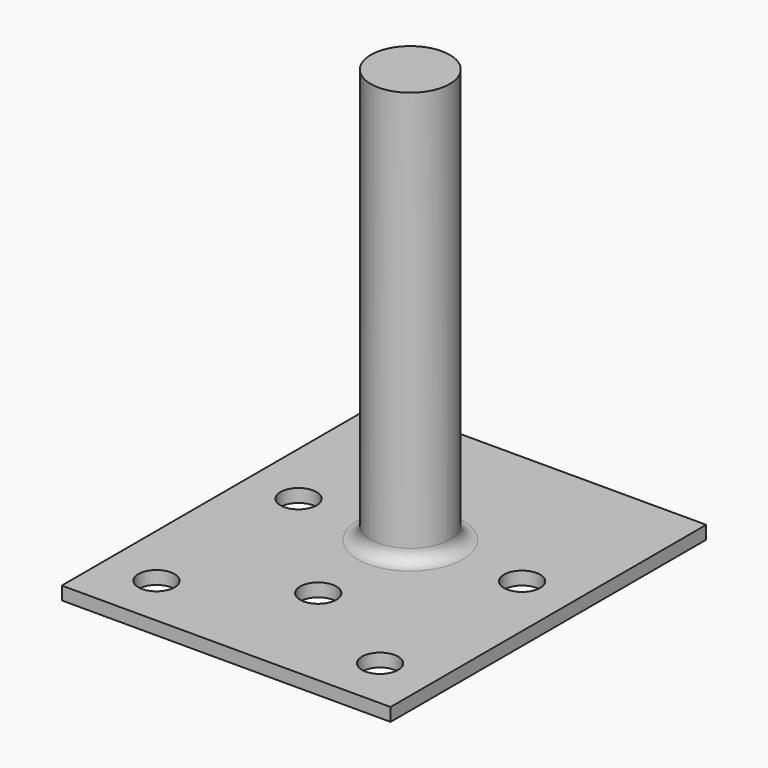
from build123d import *

# Parameters (mm, degrees)
F0_R     = 5.5
F0_R_2   = 12
F1_DEPTH = 4
F2_R     = 12
F3_DEPTH = 130
F4_R     = 4


with BuildPart() as f1:
    # F0 (on Top) → F1 (new body)
    with BuildSketch(Plane.XY):
        Polygon((50, 50), (0, 50), (-50, 50), (-50, -70), (0, -70), (50, -70), align=None)
        with Locations((-34, -54)):
            Circle(F0_R, mode=Mode.SUBTRACT)
        with Locations((34, -54)):
            Circle(F0_R, mode=Mode.SUBTRACT)
        with Locations((0, -35)):
            Circle(F0_R, mode=Mode.SUBTRACT)
        with Locations((-34, 0)):
            Circle(F0_R, mode=Mode.SUBTRACT)
        Circle(F0_R_2, mode=Mode.SUBTRACT)
        with Locations((34, 0)):
            Circle(F0_R, mode=Mode.SUBTRACT)
    extrude(amount=F1_DEPTH)

    # F2 (on face) → F3 (join)
    with BuildSketch(Plane(origin=(0, 0, 0), x_dir=(1, 0, 0), z_dir=(0, 0, -1))):
        Circle(F2_R)
    extrude(amount=-F3_DEPTH)

    # F4
    f4_edges = [f1.edges().sort_by_distance(p)[0] for p in [
        (-12, 0, 4),
    ]]
    fillet(f4_edges, radius=F4_R)


solid = f1.part
